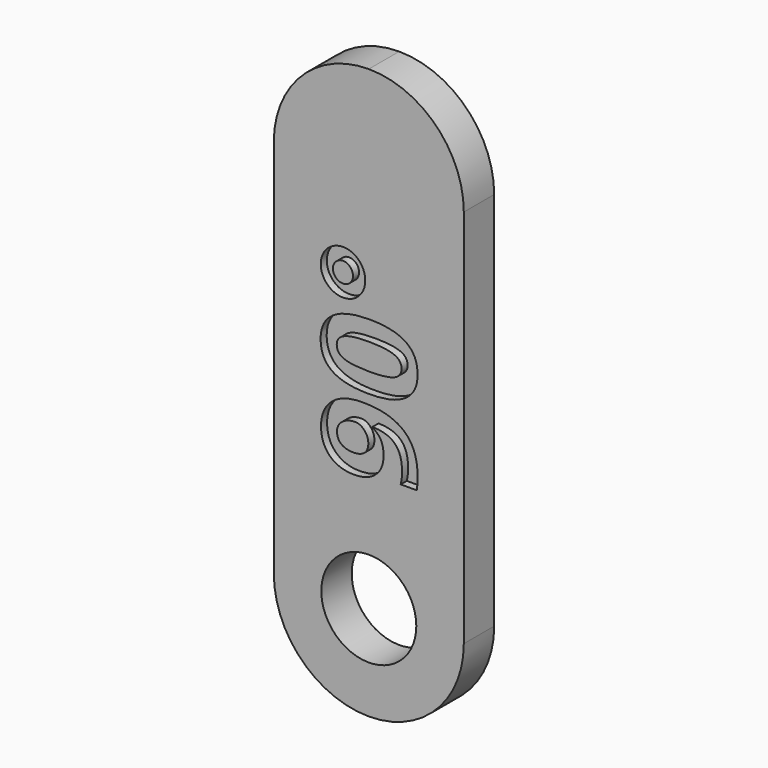
from build123d import *

# Parameters (mm, degrees)
F0_W         = 12.7
F0_H         = 38.1
F0_R         = 3.175
F1_DEPTH     = 2.54
F2_R         = 6.34999
F3_TEXT_SIZE = 8.8194444444
F4_DEPTH     = 0.508


# Not quite as in the source:
# - a fillet or chamfer is up to 0.001 mm smaller than in the source, because OpenCascade refuses the exact size
# - Text() gives the source's letters only with a copy of the font that has no kerning and outlines rounded to 1/6400 em; it was checked with that copy


with BuildPart() as f1:
    # F0 (on Front) → F1 (new body)
    with BuildSketch(Plane.XZ):
        with Locations((6.35, 19.05)):
            Rectangle(F0_W, F0_H)
        with Locations((6.35, 6.35)):
            Circle(F0_R, mode=Mode.SUBTRACT)
    extrude(amount=F1_DEPTH)

    # F2 (radius 6.35 in the source; OpenCascade refuses exactly that, so slightly less here)
    f2_edges = [f1.edges().sort_by_distance(p)[0] for p in [
        (12.7, -1.27, 0),
        (0, -1.27, 0),
        (12.7, -1.27, 38.1),
        (0, -1.27, 38.1),
    ]]
    fillet(f2_edges, radius=F2_R)

    # F3 (on face) → F4 (cut)
    with BuildSketch(Plane.XZ.offset(2.54)):
        with Locations(Location((9.525, 13.6294867622), (0, 0, 90))):
            Text('90°', F3_TEXT_SIZE, font='Open Sans', font_style=FontStyle.BOLD, text_align=(TextAlign.LEFT, TextAlign.BOTTOM))
    extrude(amount=-F4_DEPTH, mode=Mode.SUBTRACT)


solid = f1.part
